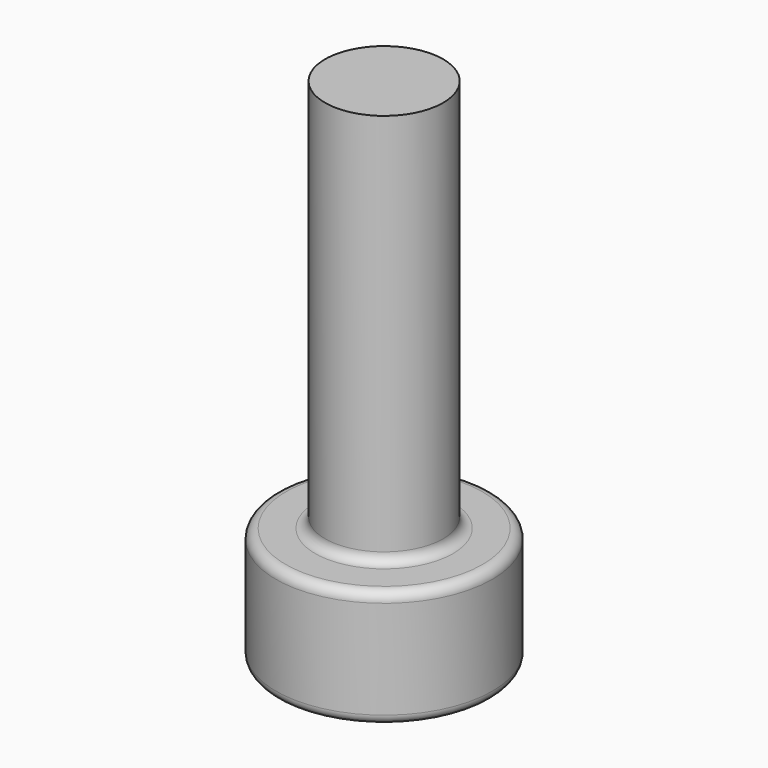
from build123d import *

# Parameters (mm, degrees)
F1_R     = 2.75
F1_R_2   = 1.5
F2_DEPTH = 3
F3_START = 1.5
F3_DEPTH = 1.5
F4_START = 3
F4_DEPTH = 10
F5_R     = 0.25


# Not quite as in the source:
# - a feature names something its author has since deleted; it is built from what else it names


with BuildPart() as f2:
    # F1 (on Top) → F2 (new body)
    with BuildSketch(Plane.XY):
        Circle(F1_R)
        Circle(F1_R_2, mode=Mode.SUBTRACT)
        Circle(F1_R_2)
        Polygon((-0.7216878365, -1.25), (-1.443375673, 0), (-0.7216878365, 1.25), (0.7216878365, 1.25), (1.443375673, 0), (0.7216878365, -1.25), align=None, mode=Mode.SUBTRACT)
    extrude(amount=F2_DEPTH)

    # F1 (on Top) → F3 (join)
    with BuildSketch(Plane.XY.offset(F3_START)):
        Polygon((-0.7216878365, 1.25), (-1.443375673, 0), (-0.7216878365, -1.25), (0.7216878365, -1.25), (1.443375673, 0), (0.7216878365, 1.25), align=None)
    extrude(amount=F3_DEPTH)

    # F1 (on Top) → F4 (join)
    with BuildSketch(Plane.XY.offset(F4_START)):
        Circle(F1_R_2)
        Polygon((-0.7216878365, -1.25), (-1.443375673, 0), (-0.7216878365, 1.25), (0.7216878365, 1.25), (1.443375673, 0), (0.7216878365, -1.25), align=None, mode=Mode.SUBTRACT)
        Polygon((-0.7216878365, 1.25), (-1.443375673, 0), (-0.7216878365, -1.25), (0.7216878365, -1.25), (1.443375673, 0), (0.7216878365, 1.25), align=None)
    extrude(amount=F4_DEPTH)

    # F5
    f5_edges = [f2.edges().sort_by_distance(p)[0] for p in [
        (-2.75, 0, 3),
        (-2.75, 0, 0),
        (-1.5, 0, 3),
    ]]
    fillet(f5_edges, radius=F5_R)


solid = f2.part
